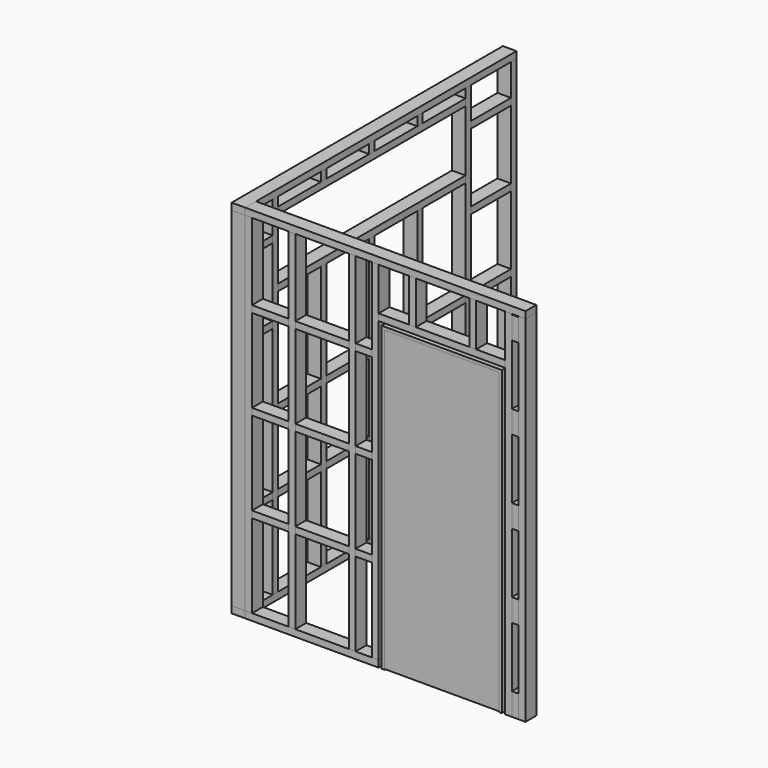
from build123d import *

# Parameters (mm, degrees)
F4_DEPTH  = 90
F3_W      = 45
F3_H      = 60
F5_DEPTH  = 90
F3_W_2    = 332.5
F3_H_2    = 45
F3_W_3    = 355
F3_W_4    = 182.5
F7_DEPTH  = 90
F6_W      = 45
F6_H      = 285
F8_DEPTH  = 90
F6_H_2    = 150
F6_W_2    = 242.5
F6_H_3    = 45
F6_W_3    = 355
F6_W_4    = 107.4999999998
F6_W_5    = 107.4999999999
F9_W      = 45
F9_H      = 90
F10_DEPTH = 2310


# Not quite as in the source:
# - ends of sketch curves that miss each other by under 0.0002 mm in the source are joined


with BuildPart() as f4:
    # F3 (on plane+point) → F4 (new body)
    with BuildSketch(Plane.YZ.offset(-1950)):
        Polygon((-45, 45), (0, 45), (0, 2355), (-45, 2355), (-45, 2145), (-45, 2100), (-45, 1645), (-45, 1600), (-45, 1145), (-45, 1100), (-45, 645), (-45, 600), align=None)
    extrude(amount=F4_DEPTH)


with BuildPart() as f4b:
    # F3 (on plane+point) → F4, piece 2 (new body)
    with BuildSketch(Plane.YZ.offset(-1950)):
        Polygon((-422.5, 45), (-377.5, 45), (-377.5, 600), (-377.5, 645), (-377.5, 1100), (-377.5, 1145), (-377.5, 1600), (-377.5, 1645), (-377.5, 2100), (-377.5, 2145), (-377.5, 2355), (-422.5, 2355), (-422.5, 2295), (-422.5, 2250), (-422.5, 1844.999833107), (-422.5, 1799.999833107), (-422.5, 1145), (-422.5, 1100), (-422.5, 645), (-422.5, 600), align=None)
    extrude(amount=F4_DEPTH)


with BuildPart() as f4c:
    # F3 (on plane+point) → F4, piece 3 (new body)
    with BuildSketch(Plane.YZ.offset(-1950)):
        with Locations((-800, 2325)):
            Rectangle(F3_W, F3_H)
    extrude(amount=F4_DEPTH)


with BuildPart() as f4d:
    # F3 (on plane+point) → F4, piece 4 (new body)
    with BuildSketch(Plane.YZ.offset(-1950)):
        with Locations((-1200, 2325)):
            Rectangle(F3_W, F3_H)
    extrude(amount=F4_DEPTH)


with BuildPart() as f4e:
    # F3 (on plane+point) → F4, piece 5 (new body)
    with BuildSketch(Plane.YZ.offset(-1950)):
        with Locations((-1600, 2325)):
            Rectangle(F3_W, F3_H)
    extrude(amount=F4_DEPTH)


with BuildPart() as f4f:
    # F3 (on plane+point) → F4, piece 6 (new body)
    with BuildSketch(Plane.YZ.offset(-1950)):
        Polygon((-2022.5, 600), (-2022.5, 45), (-1977.5, 45), (-1977.5, 600), (-1977.5, 645), (-1977.5, 1100), (-1977.5, 1145), (-1977.5, 1799.999833107), (-1977.5, 1844.999833107), (-1977.5, 2250), (-1977.5, 2295), (-1977.5, 2355), (-2022.5, 2355), (-2022.5, 2145), (-2022.5, 2100), (-2022.5, 1645), (-2022.5, 1600), (-2022.5, 1145), (-2022.5, 1100), (-2022.5, 645), align=None)
    extrude(amount=F4_DEPTH)


with BuildPart() as f4g:
    # F3 (on plane+point) → F4, piece 7 (new body)
    with BuildSketch(Plane.YZ.offset(-1950)):
        Polygon((-2250, 2355), (-2250, 45), (-2205, 45), (-2205, 600), (-2205, 645), (-2205, 1100), (-2205, 1145), (-2205, 1600), (-2205, 1645), (-2205, 2100), (-2205, 2145), (-2205, 2355), align=None)
    extrude(amount=F4_DEPTH)


with BuildPart() as f4h:
    # F3 (on plane+point) → F4, piece 8 (new body)
    with BuildSketch(Plane.YZ.offset(-1950)):
        Polygon((-1622.5, 600), (-1622.5, 45), (-1577.5, 45), (-1577.5, 600), (-1577.5, 645), (-1577.5, 1100), (-1577.5, 1145), (-1577.5, 1799.999833107), (-1622.5, 1799.999833107), (-1622.5, 1145), (-1622.5, 1100), (-1622.5, 645), align=None)
    extrude(amount=F4_DEPTH)


with BuildPart() as f4i:
    # F3 (on plane+point) → F4, piece 9 (new body)
    with BuildSketch(Plane.YZ.offset(-1950)):
        Polygon((-1222.5, 45), (-1177.5, 45), (-1177.5, 600), (-1177.5, 645), (-1177.5, 1100), (-1177.5, 1145), (-1177.5, 1799.999833107), (-1222.5, 1799.999833107), (-1222.5, 1145), (-1222.5, 1100), (-1222.5, 645), (-1222.5, 600), align=None)
    extrude(amount=F4_DEPTH)


with BuildPart() as f4j:
    # F3 (on plane+point) → F4, piece 10 (new body)
    with BuildSketch(Plane.YZ.offset(-1950)):
        Polygon((-822.5, 45), (-777.5, 45), (-777.5, 600), (-777.5, 645), (-777.5, 1100), (-777.5, 1145), (-777.5, 1799.999833107), (-822.5, 1799.999833107), (-822.5, 1145), (-822.5, 1100), (-822.5, 645), (-822.5, 600), align=None)
    extrude(amount=F4_DEPTH)


with BuildPart() as f5:
    # F3 (on plane+point) → F5 (new body)
    with BuildSketch(Plane.YZ.offset(-1950)):
        Polygon((-45, 2355), (0, 2355), (0, 2400), (-2250, 2400), (-2250, 2355), (-2205, 2355), (-2022.5, 2355), (-1977.5, 2355), (-1622.5, 2355), (-1577.5, 2355), (-1222.5, 2355), (-1177.5, 2355), (-822.5, 2355), (-777.5, 2355), (-422.5, 2355), (-377.5, 2355), align=None)
    extrude(amount=F5_DEPTH)


with BuildPart() as f5b:
    # F3 (on plane+point) → F5, piece 2 (new body)
    with BuildSketch(Plane.YZ.offset(-1950)):
        Polygon((-422.5, 2250), (-422.5, 2295), (-777.5, 2295), (-822.5, 2295), (-1177.5, 2295), (-1222.5, 2295), (-1577.5, 2295), (-1622.5, 2295), (-1977.5, 2295), (-1977.5, 2250), align=None)
    extrude(amount=F5_DEPTH)


with BuildPart() as f5c:
    # F3 (on plane+point) → F5, piece 3 (new body)
    with BuildSketch(Plane.YZ.offset(-1950)):
        with Locations((-211.25, 2122.5)):
            Rectangle(F3_W_2, F3_H_2)
    extrude(amount=F5_DEPTH)


with BuildPart() as f5d:
    # F3 (on plane+point) → F5, piece 4 (new body)
    with BuildSketch(Plane.YZ.offset(-1950)):
        Polygon((-422.5, 1799.999833107), (-422.5, 1844.999833107), (-1977.5, 1844.999833107), (-1977.5, 1799.999833107), (-1622.5, 1799.999833107), (-1577.5, 1799.999833107), (-1222.5, 1799.999833107), (-1177.5, 1799.999833107), (-822.5, 1799.999833107), (-777.5, 1799.999833107), align=None)
    extrude(amount=F5_DEPTH)


with BuildPart() as f5e:
    # F3 (on plane+point) → F5, piece 5 (new body)
    with BuildSketch(Plane.YZ.offset(-1950)):
        with Locations((-211.25, 1622.5)):
            Rectangle(F3_W_2, F3_H_2)
    extrude(amount=F5_DEPTH)


with BuildPart() as f5f:
    # F3 (on plane+point) → F5, piece 6 (new body)
    with BuildSketch(Plane.YZ.offset(-1950)):
        with Locations((-211.25, 1122.5)):
            Rectangle(F3_W_2, F3_H_2)
    extrude(amount=F5_DEPTH)


with BuildPart() as f5g:
    # F3 (on plane+point) → F5, piece 7 (new body)
    with BuildSketch(Plane.YZ.offset(-1950)):
        with Locations((-600, 1122.5)):
            Rectangle(F3_W_3, F3_H_2)
    extrude(amount=F5_DEPTH)


with BuildPart() as f5h:
    # F3 (on plane+point) → F5, piece 8 (new body)
    with BuildSketch(Plane.YZ.offset(-1950)):
        with Locations((-1000, 1122.5)):
            Rectangle(F3_W_3, F3_H_2)
    extrude(amount=F5_DEPTH)


with BuildPart() as f5i:
    # F3 (on plane+point) → F5, piece 9 (new body)
    with BuildSketch(Plane.YZ.offset(-1950)):
        with Locations((-1400, 1122.5)):
            Rectangle(F3_W_3, F3_H_2)
    extrude(amount=F5_DEPTH)


with BuildPart() as f5j:
    # F3 (on plane+point) → F5, piece 10 (new body)
    with BuildSketch(Plane.YZ.offset(-1950)):
        with Locations((-1800, 1122.5)):
            Rectangle(F3_W_3, F3_H_2)
    extrude(amount=F5_DEPTH)


with BuildPart() as f5k:
    # F3 (on plane+point) → F5, piece 11 (new body)
    with BuildSketch(Plane.YZ.offset(-1950)):
        with Locations((-2113.75, 1122.5)):
            Rectangle(F3_W_4, F3_H_2)
    extrude(amount=F5_DEPTH)


with BuildPart() as f5l:
    # F3 (on plane+point) → F5, piece 12 (new body)
    with BuildSketch(Plane.YZ.offset(-1950)):
        with Locations((-2113.75, 622.5)):
            Rectangle(F3_W_4, F3_H_2)
    extrude(amount=F5_DEPTH)


with BuildPart() as f5m:
    # F3 (on plane+point) → F5, piece 13 (new body)
    with BuildSketch(Plane.YZ.offset(-1950)):
        with Locations((-1800, 622.5)):
            Rectangle(F3_W_3, F3_H_2)
    extrude(amount=F5_DEPTH)


with BuildPart() as f5n:
    # F3 (on plane+point) → F5, piece 14 (new body)
    with BuildSketch(Plane.YZ.offset(-1950)):
        with Locations((-1400, 622.5)):
            Rectangle(F3_W_3, F3_H_2)
    extrude(amount=F5_DEPTH)


with BuildPart() as f5o:
    # F3 (on plane+point) → F5, piece 15 (new body)
    with BuildSketch(Plane.YZ.offset(-1950)):
        with Locations((-1000, 622.5)):
            Rectangle(F3_W_3, F3_H_2)
    extrude(amount=F5_DEPTH)


with BuildPart() as f5p:
    # F3 (on plane+point) → F5, piece 16 (new body)
    with BuildSketch(Plane.YZ.offset(-1950)):
        with Locations((-600, 622.5)):
            Rectangle(F3_W_3, F3_H_2)
    extrude(amount=F5_DEPTH)


with BuildPart() as f5q:
    # F3 (on plane+point) → F5, piece 17 (new body)
    with BuildSketch(Plane.YZ.offset(-1950)):
        with Locations((-211.25, 622.5)):
            Rectangle(F3_W_2, F3_H_2)
    extrude(amount=F5_DEPTH)


with BuildPart() as f5r:
    # F3 (on plane+point) → F5, piece 18 (new body)
    with BuildSketch(Plane.YZ.offset(-1950)):
        Polygon((-2250, 0), (0, 0), (0, 45), (-45, 45), (-377.5, 45), (-422.5, 45), (-777.5, 45), (-822.5, 45), (-1177.5, 45), (-1222.5, 45), (-1577.5, 45), (-1622.5, 45), (-1977.5, 45), (-2022.5, 45), (-2205, 45), (-2250, 45), align=None)
    extrude(amount=F5_DEPTH)


with BuildPart() as f5s:
    # F3 (on plane+point) → F5, piece 19 (new body)
    with BuildSketch(Plane.YZ.offset(-1950)):
        with Locations((-2113.75, 1622.5)):
            Rectangle(F3_W_4, F3_H_2)
    extrude(amount=F5_DEPTH)


with BuildPart() as f5t:
    # F3 (on plane+point) → F5, piece 20 (new body)
    with BuildSketch(Plane.YZ.offset(-1950)):
        with Locations((-2113.75, 2122.5)):
            Rectangle(F3_W_4, F3_H_2)
    extrude(amount=F5_DEPTH)


with BuildPart() as f7:
    # F6 (on plane+point) → F7 (new body)
    with BuildSketch(Plane.XZ.offset(2250)):
        Polygon((-1815, 2355), (-1860, 2355), (-1860, 45), (-1815, 45), (-1815, 600), (-1815, 645), (-1815, 1200), (-1815, 1245), (-1815, 1800), (-1815, 1845), align=None)
    extrude(amount=-F7_DEPTH)


with BuildPart() as f7b:
    # F6 (on plane+point) → F7, piece 2 (new body)
    with BuildSketch(Plane.XZ.offset(2250)):
        Polygon((-1527.5, 2355), (-1572.5, 2355), (-1572.5, 1845), (-1572.5, 1800), (-1572.5, 1245), (-1572.5, 1200), (-1572.5, 645), (-1572.5, 600), (-1572.5, 45), (-1527.5, 45), (-1527.5, 600), (-1527.5, 645), (-1527.5, 1200), (-1527.5, 1245), (-1527.5, 1800), (-1527.5, 1845), align=None)
    extrude(amount=-F7_DEPTH)


with BuildPart() as f7c:
    # F6 (on plane+point) → F7, piece 3 (new body)
    with BuildSketch(Plane.XZ.offset(2250)):
        Polygon((-1127.5, 2355), (-1172.5, 2355), (-1172.5, 1845), (-1172.5, 1800), (-1172.5, 1245), (-1172.5, 1200), (-1172.5, 645), (-1172.5, 600), (-1172.5, 45), (-1127.4999999998, 45), (-1127.4999999998, 600), (-1127.4999999998, 645), (-1127.4999999999, 1200), (-1127.4999999999, 1245), (-1127.4999999999, 1800), (-1127.4999999999, 1845), align=None)
    extrude(amount=-F7_DEPTH)


with BuildPart() as f7d:
    # F6 (on plane+point) → F7, piece 4 (new body)
    with BuildSketch(Plane.XZ.offset(2250)):
        with Locations((-750, 2212.5)):
            Rectangle(F6_W, F6_H)
    extrude(amount=-F7_DEPTH)


with BuildPart() as f7e:
    # F6 (on plane+point) → F7, piece 5 (new body)
    with BuildSketch(Plane.XZ.offset(2250)):
        with Locations((-350, 2212.5)):
            Rectangle(F6_W, F6_H)
    extrude(amount=-F7_DEPTH)


with BuildPart() as f7f:
    # F6 (on plane+point) → F7, piece 6 (new body)
    with BuildSketch(Plane.XZ.offset(2250)):
        Polygon((-90, 2350), (-90, 2355), (-135, 2355), (-135, 2070), (-135, 2025), (-135, 45.5069230115), (-135, 0), (-90, 0), (-90, 150), (-90, 550), (-90, 700), (-90, 1100), (-90, 1250), (-90, 1650), (-90, 1800), (-90, 2200), align=None)
    extrude(amount=-F7_DEPTH)


with BuildPart() as f7g:
    # F6 (on plane+point) → F7, piece 7 (new body)
    with BuildSketch(Plane.XZ.offset(2250)):
        Polygon((0, 0), (0, 2355), (-45, 2355), (-45, 2350), (-45, 2200), (-45, 1800), (-45, 1650), (-45, 1250), (-45, 1100), (-45, 700), (-45, 550), (-45, 150), (-45, 0), align=None)
    extrude(amount=-F7_DEPTH)


with BuildPart() as f7h:
    # F6 (on plane+point) → F7, piece 8 (new body)
    with BuildSketch(Plane.XZ.offset(2250)):
        Polygon((-1020, 45), (-975, 45), (-975, 2025), (-975, 2070), (-975, 2355), (-1020, 2355), (-1020, 1845), (-1020, 1800), (-1020, 1245), (-1020, 1200), (-1020, 645), (-1020, 600), align=None)
    extrude(amount=-F7_DEPTH)


with BuildPart() as f7i:
    # F6 (on plane+point) → F7, piece 9 (new body)
    with BuildSketch(Plane.XZ.offset(2250)):
        Polygon((-175, 5), (-175, 45), (-175, 1985), (-935, 1985), (-935, 45), (-935, 5), align=None)
    extrude(amount=-F7_DEPTH)


with BuildPart() as f8:
    # F6 (on plane+point) → F8 (new body)
    with BuildSketch(Plane.XZ.offset(2250)):
        Polygon((0, 2400), (-1860, 2400), (-1860, 2355), (-1815, 2355), (-1572.5, 2355), (-1527.5, 2355), (-1172.5, 2355), (-1127.5, 2355), (-1020, 2355), (-975, 2355), (-772.5, 2355), (-727.5, 2355), (-372.5, 2355), (-327.5, 2355), (-135, 2355), (-90, 2355), (-45, 2355), (0, 2355), align=None)
    extrude(amount=-F8_DEPTH)


with BuildPart() as f8b:
    # F6 (on plane+point) → F8, piece 2 (new body)
    with BuildSketch(Plane.XZ.offset(2250)):
        Polygon((-135, 2025), (-135, 2070), (-327.5, 2070), (-372.5, 2070), (-727.5, 2070), (-772.5, 2070), (-975, 2070), (-975, 2025), align=None)
    extrude(amount=-F8_DEPTH)


with BuildPart() as f8c:
    # F6 (on plane+point) → F8, piece 3 (new body)
    with BuildSketch(Plane.XZ.offset(2250)):
        Polygon((-1815, 45), (-1860, 45), (-1860, 0), (-975, 0), (-975, 45), (-1020, 45), (-1127.4999999998, 45), (-1172.5, 45), (-1527.5, 45), (-1572.5, 45), align=None)
    extrude(amount=-F8_DEPTH)


with BuildPart() as f8d:
    # F6 (on plane+point) → F8, piece 4 (new body)
    with BuildSketch(Plane.XZ.offset(2250)):
        with Locations((-67.5, 2275)):
            Rectangle(F6_W, F6_H_2)
    extrude(amount=-F8_DEPTH)


with BuildPart() as f8e:
    # F6 (on plane+point) → F8, piece 5 (new body)
    with BuildSketch(Plane.XZ.offset(2250)):
        with Locations((-67.5, 1725)):
            Rectangle(F6_W, F6_H_2)
    extrude(amount=-F8_DEPTH)


with BuildPart() as f8f:
    # F6 (on plane+point) → F8, piece 6 (new body)
    with BuildSketch(Plane.XZ.offset(2250)):
        with Locations((-67.5, 1175)):
            Rectangle(F6_W, F6_H_2)
    extrude(amount=-F8_DEPTH)


with BuildPart() as f8g:
    # F6 (on plane+point) → F8, piece 7 (new body)
    with BuildSketch(Plane.XZ.offset(2250)):
        with Locations((-67.5, 625)):
            Rectangle(F6_W, F6_H_2)
    extrude(amount=-F8_DEPTH)


with BuildPart() as f8h:
    # F6 (on plane+point) → F8, piece 8 (new body)
    with BuildSketch(Plane.XZ.offset(2250)):
        with Locations((-67.5, 75)):
            Rectangle(F6_W, F6_H_2)
    extrude(amount=-F8_DEPTH)


with BuildPart() as f8i:
    # F6 (on plane+point) → F8, piece 9 (new body)
    with BuildSketch(Plane.XZ.offset(2250)):
        with Locations((-1693.75, 622.5)):
            Rectangle(F6_W_2, F6_H_3)
    extrude(amount=-F8_DEPTH)


with BuildPart() as f8j:
    # F6 (on plane+point) → F8, piece 10 (new body)
    with BuildSketch(Plane.XZ.offset(2250)):
        with Locations((-1350, 622.5)):
            Rectangle(F6_W_3, F6_H_3)
    extrude(amount=-F8_DEPTH)


with BuildPart() as f8k:
    # F6 (on plane+point) → F8, piece 11 (new body)
    with BuildSketch(Plane.XZ.offset(2250)):
        with Locations((-1073.7499999999, 622.5)):
            Rectangle(F6_W_4, F6_H_3)
    extrude(amount=-F8_DEPTH)


with BuildPart() as f8l:
    # F6 (on plane+point) → F8, piece 12 (new body)
    with BuildSketch(Plane.XZ.offset(2250)):
        with Locations((-1073.7499999999, 1222.5)):
            Rectangle(F6_W_5, F6_H_3)
    extrude(amount=-F8_DEPTH)


with BuildPart() as f8m:
    # F6 (on plane+point) → F8, piece 13 (new body)
    with BuildSketch(Plane.XZ.offset(2250)):
        with Locations((-1350, 1222.5)):
            Rectangle(F6_W_3, F6_H_3)
    extrude(amount=-F8_DEPTH)


with BuildPart() as f8n:
    # F6 (on plane+point) → F8, piece 14 (new body)
    with BuildSketch(Plane.XZ.offset(2250)):
        with Locations((-1693.75, 1222.5)):
            Rectangle(F6_W_2, F6_H_3)
    extrude(amount=-F8_DEPTH)


with BuildPart() as f8o:
    # F6 (on plane+point) → F8, piece 15 (new body)
    with BuildSketch(Plane.XZ.offset(2250)):
        with Locations((-1693.75, 1822.5)):
            Rectangle(F6_W_2, F6_H_3)
    extrude(amount=-F8_DEPTH)


with BuildPart() as f8p:
    # F6 (on plane+point) → F8, piece 16 (new body)
    with BuildSketch(Plane.XZ.offset(2250)):
        with Locations((-1350, 1822.5)):
            Rectangle(F6_W_3, F6_H_3)
    extrude(amount=-F8_DEPTH)


with BuildPart() as f8q:
    # F6 (on plane+point) → F8, piece 17 (new body)
    with BuildSketch(Plane.XZ.offset(2250)):
        with Locations((-1073.75, 1822.5)):
            Rectangle(F6_W_5, F6_H_3)
    extrude(amount=-F8_DEPTH)


with BuildPart() as f8r:
    # F6 (on plane+point) → F8, piece 18 (new body)
    with BuildSketch(Plane.XZ.offset(2250)):
        Polygon((-175, 1985), (-175, 45), (-175, 5), (-175, 0), (-156.86622262, 0), (-156.86622262, 2005), (-955, 2005), (-955, 0), (-935, 0), (-935, 5), (-935, 45), (-935, 1985), align=None)
    extrude(amount=-F8_DEPTH)


with BuildPart() as f10:
    # F9 (on face) → F10 (new body, through all)
    with BuildSketch(Plane.XY.offset(45)):
        with Locations((-1882.5, -2160)):
            Rectangle(F9_W, F9_H)
    extrude(amount=F10_DEPTH)

    # F11: cut F5t, F5s, F5k, F5l
    add(f5t.part, mode=Mode.SUBTRACT)
    add(f5s.part, mode=Mode.SUBTRACT)
    add(f5k.part, mode=Mode.SUBTRACT)
    add(f5l.part, mode=Mode.SUBTRACT)


solid = Compound([f4.part, f4b.part, f4c.part, f4d.part, f4e.part, f4f.part, f4g.part, f4h.part, f4i.part, f4j.part, f5.part, f5b.part, f5c.part, f5d.part, f5e.part, f5f.part, f5g.part, f5h.part, f5i.part, f5j.part, f5k.part, f5l.part, f5m.part, f5n.part, f5o.part, f5p.part, f5q.part, f5r.part, f5s.part, f5t.part, f7.part, f7b.part, f7c.part, f7d.part, f7e.part, f7f.part, f7g.part, f7h.part, f7i.part, f8.part, f8b.part, f8c.part, f8d.part, f8e.part, f8f.part, f8g.part, f8h.part, f8i.part, f8j.part, f8k.part, f8l.part, f8m.part, f8n.part, f8o.part, f8p.part, f8q.part, f8r.part, f10.part])
